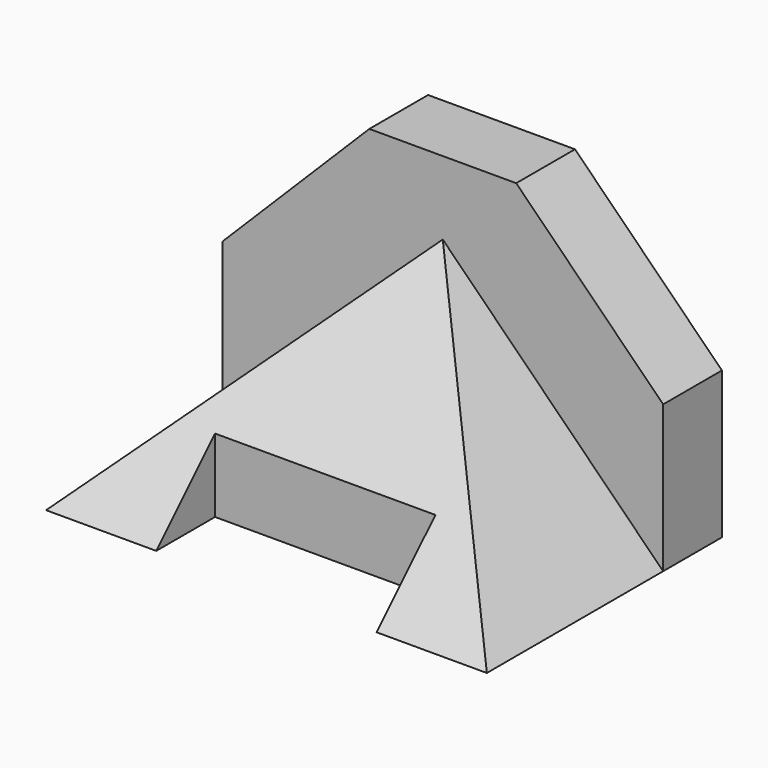
from build123d import *

# Parameters (mm, degrees)
F1_DEPTH = 76.2
F3_DEPTH = 38.1
F5_DEPTH = 12.701
F6_W     = 38.1
F6_H     = 12.7
F7_DEPTH = 12.7


with BuildPart() as f1:
    # F0 (on Right) → F1 (new body)
    with BuildSketch(Plane.YZ):
        Polygon((38.1, 38.1), (0, 0), (38.1, 0), align=None)
        Polygon((38.1, 38.1), (38.1, 0), (50.8, 0), (50.8, 50.8), (38.1, 50.8), align=None)
    extrude(amount=F1_DEPTH)

    # F2 (on Front) → F3 (cut, through all)
    with BuildSketch(Plane.XZ):
        Polygon((76.2, 38.1), (38.1, 38.1), (76.2, 0), align=None)
        Polygon((0, 38.1), (0, 0), (38.1, 38.1), align=None)
    extrude(amount=-F3_DEPTH, mode=Mode.SUBTRACT)

    # F4 (on face) → F5 (cut, through all)
    with BuildSketch(Plane.XZ.offset(-38.1)):
        Polygon((25.4, 50.8), (0, 50.8), (0, 25.4), align=None)
        Polygon((76.2, 50.8), (50.8, 50.8), (76.2, 25.4), align=None)
    extrude(amount=-F5_DEPTH, mode=Mode.SUBTRACT)

    # F6 (on Front) → F7 (cut)
    with BuildSketch(Plane.XZ):
        with Locations((38.1, 6.35)):
            Rectangle(F6_W, F6_H)
    extrude(amount=-F7_DEPTH, mode=Mode.SUBTRACT)


solid = f1.part
